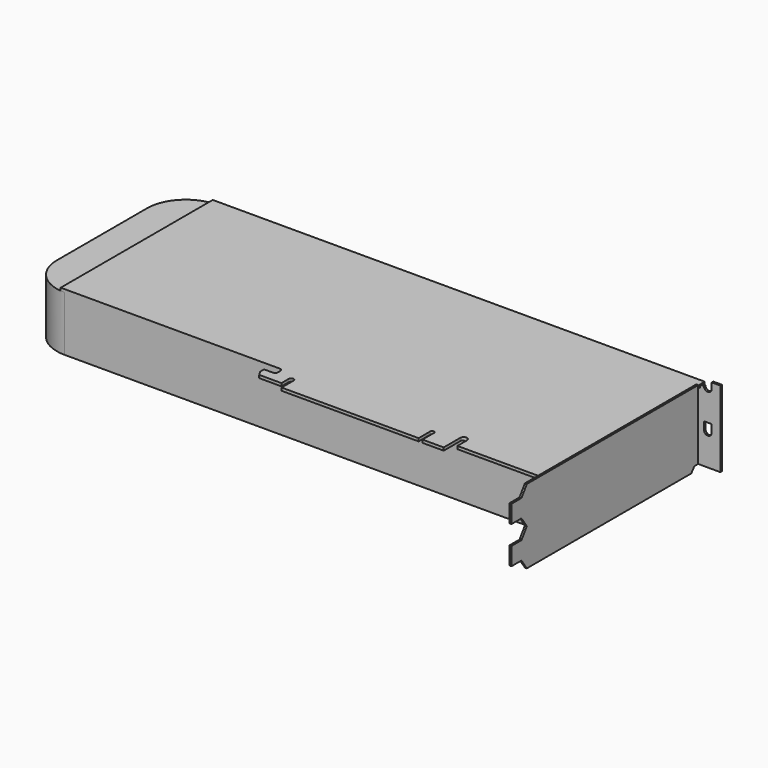
from build123d import *

# Parameters (mm, degrees)
F1_DEPTH  = 1.5
F3_DEPTH  = 1
F4_R      = 0.99999
F5_R      = 1.74999
F6_R      = 1.24999
F7_R      = 1.5
F9_DEPTH  = 1
F11_DEPTH = 33.5
F12_SIZE2 = 5
F12_SIZE  = 18.6602540378


# Not quite as in the source:
# - a fillet or chamfer is up to 0.001 mm smaller than in the source, because OpenCascade refuses the exact size


with BuildPart() as f1:
    # F0 (on Top) → F1 (new body)
    with BuildSketch(Plane.XY):
        Polygon((84.5, -53.25), (127.5, -53.25), (127.5, 53.25), (-127.5, 53.25), (-127.5, -45.25), (-12.5, -45.25), (-12.5, -49.75), (-18.5, -49.75), (-18.5, -52.25), (-17, -54.75), (-5.5, -54.75), (-5.5, -48.75), (-3, -48.75), (-3, -57.75), (68, -57.75), (68, -49.25), (70, -49.25), (70, -57.75), (81, -57.75), (81, -45.25), (84.5, -45.25), align=None)
    extrude(amount=F1_DEPTH)

    # F2 (on face) → F3 (join)
    with BuildSketch(Plane.YZ.offset(127.5)):
        Polygon((47.75, 2.5), (-63.25, 2.5), (-66.75, -2.5), (-73.25, -2.5), (-73.25, -11.75), (-66.75, -11.75), (-63.25, -16.75), (-66.75, -21.75), (-73.25, -21.75), (-73.25, -31), (-66.75, -31), (-63.25, -36), (43.25, -36), (45.25, -33.5), (47.75, -33.5), align=None)
    extrude(amount=F3_DEPTH)

    # F4 (radius 1 in the source; OpenCascade refuses exactly that, so slightly less here)
    f4_edges = [f1.edges().sort_by_distance(p)[0] for p in [
        (68, -49.25, 0.75),
        (70, -49.25, 0.75),
    ]]
    fillet(f4_edges, radius=F4_R)

    # F5 (radius 1.75 in the source; OpenCascade refuses exactly that, so slightly less here)
    f5_edges = [f1.edges().sort_by_distance(p)[0] for p in [
        (81, -45.25, 0.75),
        (84.5, -45.25, 0.75),
    ]]
    fillet(f5_edges, radius=F5_R)

    # F6 (radius 1.25 in the source; OpenCascade refuses exactly that, so slightly less here)
    f6_edges = [f1.edges().sort_by_distance(p)[0] for p in [
        (-5.5, -48.75, 0.75),
        (-3, -48.75, 0.75),
    ]]
    fillet(f6_edges, radius=F6_R)

    # F7
    f7_edges = [f1.edges().sort_by_distance(p)[0] for p in [
        (-12.5, -49.75, 0.75),
        (-12.5, -45.25, 0.75),
    ]]
    fillet(f7_edges, radius=F7_R)

    # F8 (on face) → F9 (join)
    with BuildSketch(Plane(origin=(0, 47.75, 0), x_dir=(-1, 0, 0), z_dir=(0, 1, 0))):
        with BuildLine():
            Line((-140, -33.5), (-127.5, -33.5))
            Line((-127.5, -33.5), (-127.5, 1.5))
            Line((-127.5, 1.5), (-129.5, 1.5))
            Line((-129.5, 1.5), (-129.5, 3))
            Line((-129.5, 3), (-131.5, 3))
            ThreePointArc((-131.5, 3), (-133.5, 1), (-135.5, 3))
            Line((-135.5, 3), (-135.5, 6))
            Line((-135.5, 6), (-140, 6))
            Line((-140, 6), (-140, -33.5))
        make_face()
        with BuildLine():
            Line((-135.5, -17), (-135.5, -13))
            Line((-135.5, -13), (-131.5, -13))
            Line((-131.5, -13), (-131.5, -17))
            ThreePointArc((-131.5, -17), (-133.5, -19), (-135.5, -17))
        make_face(mode=Mode.SUBTRACT)
    extrude(amount=F9_DEPTH)

    # F10 (on face) → F11 (join, through all)
    with BuildSketch(Plane(origin=(0, 0, 0), x_dir=(1, 0, 0), z_dir=(0, 0, -1))):
        with BuildLine():
            Line((126.5, -53.25), (126.5, 45.25))
            Line((126.5, 45.25), (-125.5, 45.25))
            ThreePointArc((-125.5, 45.25), (-139.6421356237, 39.3921356237), (-145.5, 25.25))
            Line((-145.5, 25.25), (-145.5, -33.25))
            ThreePointArc((-145.5, -33.25), (-139.6421356237, -47.3921356237), (-125.5, -53.25))
            Line((-125.5, -53.25), (126.5, -53.25))
        make_face()
    extrude(amount=F11_DEPTH)

    # F12
    f12_edges = [f1.edges().sort_by_distance(p)[0] for p in [
        (0.5, -45.25, -33.5),
        (0.5, 53.25, -33.5),
    ]]
    f12_side = f1.faces().sort_by_distance((-8.651711, 4, -33.5))[0]
    chamfer(f12_edges, length=F12_SIZE, length2=F12_SIZE2, reference=f12_side)


solid = f1.part
